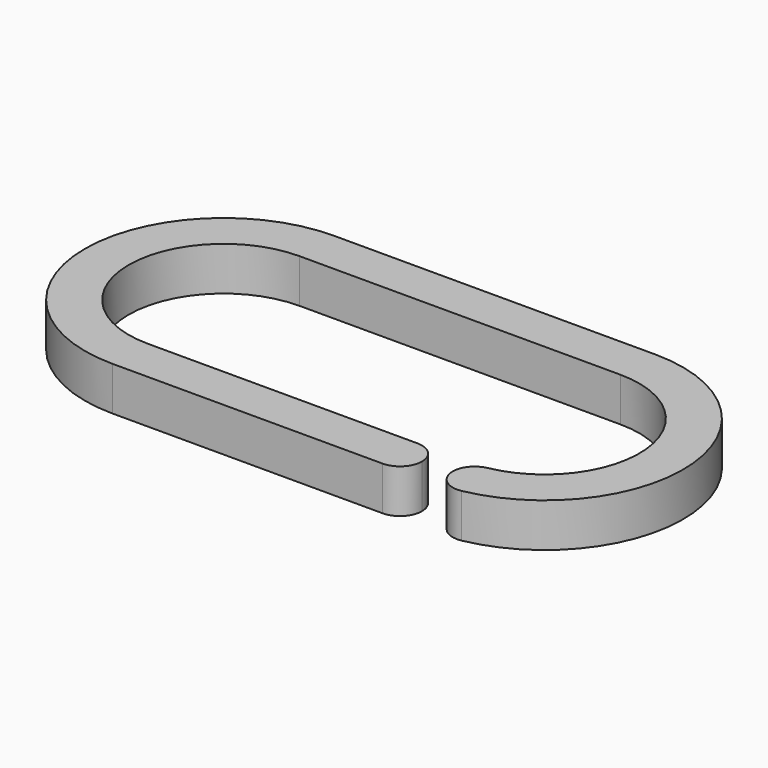
from build123d import *

# Parameters (mm, degrees)
F1_DEPTH = 3
F2_R     = 1.49999


# Not quite as in the source:
# - a fillet or chamfer is up to 0.001 mm smaller than in the source, because OpenCascade refuses the exact size


with BuildPart() as f1:
    # F0 (on Top) → F1 (new body)
    with BuildSketch(Plane.XY):
        with BuildLine():
            ThreePointArc((0, -6.5), (-6.5, 0), (0, 6.5))
            Line((0, 6.5), (22, 6.5))
            ThreePointArc((22, 6.5), (28.5, 0), (22, -6.5))
            Line((22, -6.5), (22, -9.5))
            ThreePointArc((22, -9.5), (31.5, 0), (22, 9.5))
            Line((22, 9.5), (0, 9.5))
            ThreePointArc((0, 9.5), (-9.5, 0), (0, -9.5))
            Line((0, -9.5), (20, -9.5))
            Line((20, -9.5), (20, -6.5))
            Line((20, -6.5), (0, -6.5))
        make_face()
    extrude(amount=F1_DEPTH)

    # F2 (radius 1.5 in the source; OpenCascade refuses exactly that, so slightly less here)
    f2_edges = [f1.edges().sort_by_distance(p)[0] for p in [
        (20, -9.5, 1.5),
        (20, -6.5, 1.5),
        (22, -6.5, 1.5),
        (22, -9.5, 1.5),
    ]]
    fillet(f2_edges, radius=F2_R)


solid = f1.part
